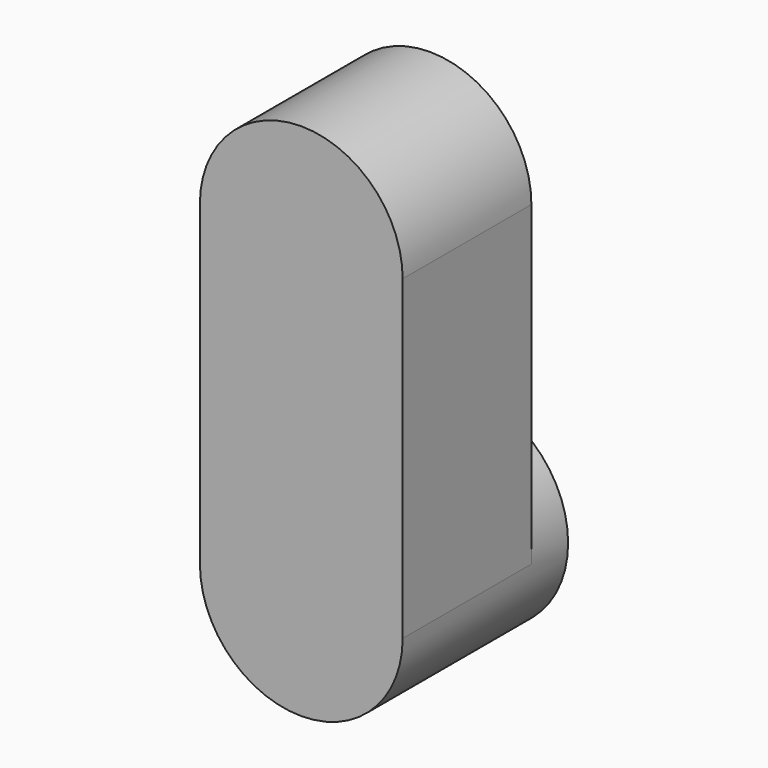
from build123d import *

# Parameters (mm, degrees)
F1_DEPTH = 7.24
F2_DEPTH = 25.4


with BuildPart() as f1:
    # F0 (on Front) → F1 (new body)
    with BuildSketch(Plane.XZ):
        with BuildLine():
            ThreePointArc((-16, -49.9569810927), (0, -65.9569810927), (16, -49.9569810927))
            ThreePointArc((16, -49.9569810927), (0, -33.9569810927), (-16, -49.9569810927))
        make_face()
    extrude(amount=-F1_DEPTH)

    # F0 (on Front) → F2 (join)
    with BuildSketch(Plane.XZ):
        with BuildLine():
            ThreePointArc((-16, 0), (0, -16), (16, 0))
            ThreePointArc((16, 0), (0, 16), (-16, 0))
        make_face()
        with BuildLine():
            Line((16, -49.9569810927), (16, 0))
            ThreePointArc((16, 0), (0, -16), (-16, 0))
            Line((-16, 0), (-16, -49.9569810927))
            ThreePointArc((-16, -49.9569810927), (0, -33.9569810927), (16, -49.9569810927))
        make_face()
        with BuildLine():
            ThreePointArc((-16, -49.9569810927), (0, -65.9569810927), (16, -49.9569810927))
            ThreePointArc((16, -49.9569810927), (0, -33.9569810927), (-16, -49.9569810927))
        make_face()
    extrude(amount=F2_DEPTH)


solid = f1.part
